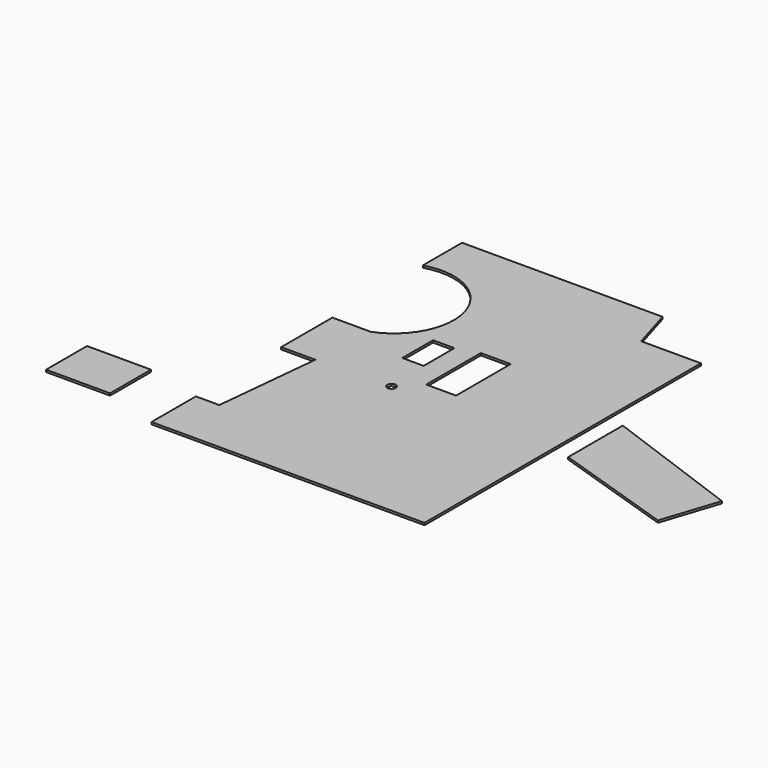
from build123d import *

# Parameters (mm, degrees)
F0_R     = 3.175
F0_W     = 22.225
F0_H     = 50.8
F0_W_2   = 15.875
F0_H_2   = 28.575
F1_DEPTH = 1.5875
F2_DEPTH = 1.5875
F0_W_3   = 47.625
F0_H_3   = 38.1
F3_DEPTH = 1.5875


# Not quite as in the source:
# - a length typed as a fraction of an inch, garbled in the dataset ("3 / 203.2 mm" for 3/8 in), is restored


with BuildPart() as f1:
    # F0 (on Top) → F1 (new body)
    with BuildSketch(Plane.XY):
        with BuildLine():
            Line((0, 0), (203.2, 0))
            Line((203.2, 0), (203.2, 257.175))
            Line((203.2, 257.175), (158.75, 257.175))
            Line((158.75, 257.175), (149.225, 288.925))
            Line((149.225, 288.925), (0, 288.925))
            Line((0, 288.925), (0, 252.4125))
            ThreePointArc((0, 252.4125), (54.7976201519, 224.0840026314), (28.5176246655, 168.275))
            Line((28.5176246655, 168.275), (0, 168.275))
            Line((0, 168.275), (0, 120.65))
            Line((0, 120.65), (25.4, 120.65))
            Line((25.4, 120.65), (17.4625, 41.275))
            Line((17.4625, 41.275), (0, 41.275))
            Line((0, 41.275), (0, 0))
        make_face()
        with Locations((80.9625, 122.2375)):
            Circle(F0_R, mode=Mode.SUBTRACT)
        with Locations((106.3625, 161.925)):
            Rectangle(F0_W, F0_H, mode=Mode.SUBTRACT)
        with Locations((71.4375, 168.275)):
            Rectangle(F0_W_2, F0_H_2, mode=Mode.SUBTRACT)
    extrude(amount=F1_DEPTH)


with BuildPart() as f2:
    # F0 (on Top) → F2 (new body)
    with BuildSketch(Plane.XY):
        Polygon((321.0547220741, 129.3808330162), (216.7015462149, 167.5800517662), (216.7015462149, 116.7800517662), (307.221789279, 87.1380529197), align=None)
    extrude(amount=F2_DEPTH)


with BuildPart() as f3:
    # F0 (on Top) → F3 (new body)
    with BuildSketch(Plane.XY):
        with Locations((-65.1747573316, 32.2102343172)):
            Rectangle(F0_W_3, F0_H_3)
    extrude(amount=F3_DEPTH)


solid = Compound([f1.part, f2.part, f3.part])
